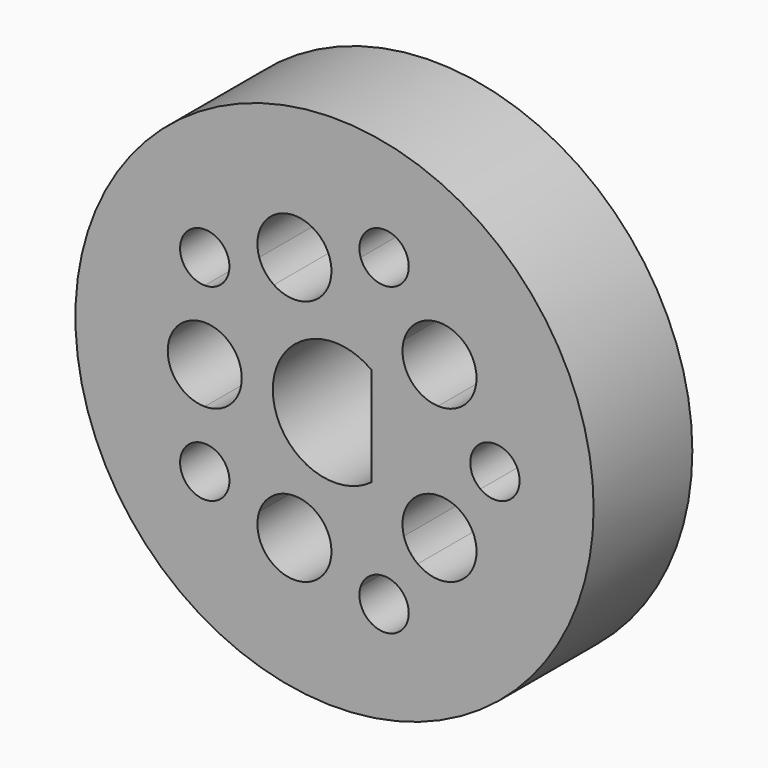
from build123d import *

# Parameters (mm, degrees)
F0_R     = 10.5
F1_DEPTH = 5


# Not quite as in the source:
# - a feature names something its author has since deleted; it is built from what else it names


with BuildPart() as f1:
    # F0 (on Front) → F1 (new body)
    with BuildSketch(Plane.XZ):
        Circle(F0_R)
        with BuildLine():
            Line((-6.1874431518, -2.6427799437), (-5.2586104634, -1.91030207))
            Line((-5.2586104634, -1.91030207), (-5.2586104634, -1.5))
            ThreePointArc((-5.2586104634, -1.5), (-6.7586104634, 0), (-5.2586104634, 1.5))
            Line((-5.2586104634, 1.5), (-5.2586104634, 1.91030207))
            Line((-5.2586104634, 1.91030207), (-6.1874431518, 2.6427799437))
            ThreePointArc((-6.1874431518, 2.6427799437), (-6.472135955, 4.7022820183), (-4.4254581722, 5.0679442137))
            Line((-4.4254581722, 5.0679442137), (-3.4418052317, 4.4109199439))
            Line((-3.4418052317, 4.4109199439), (-3.0515847744, 4.5377102563))
            ThreePointArc((-3.0515847744, 4.5377102563), (-2.0885254916, 6.4278205224), (-0.1984152256, 5.4647612395))
            Line((-0.1984152256, 5.4647612395), (0.1918052317, 5.5915515519))
            Line((0.1918052317, 5.5915515519), (0.601408001, 6.7012720437))
            ThreePointArc((0.601408001, 6.7012720437), (2.2724250824, 7.6584857382), (3.5086104634, 6.1818673559))
            ThreePointArc((3.5086104634, 6.1818673559), (3.4944811986, 5.976469794), (3.4523595855, 5.7749417209))
            Line((3.4523595855, 5.7749417209), (3.1314578476, 4.6364005169))
            Line((3.1314578476, 4.6364005169), (3.3726273533, 4.3044591695))
            ThreePointArc((3.3726273533, 4.3044591695), (4.9352909813, 4.4274434642), (5.7543052317, 3.090933678))
            ThreePointArc((5.7543052317, 3.090933678), (5.590815018, 2.4099479283), (5.1359831102, 1.8774081864))
            Line((5.1359831102, 1.8774081864), (5.3771526159, 1.545466839))
            Line((5.3771526159, 1.545466839), (6.5591337375, 1.4988339471))
            ThreePointArc((6.5591337375, 1.4988339471), (7.5813650184, 1.0395430231), (8, 0))
            ThreePointArc((8, 0), (7.5813650184, -1.0395430231), (6.5591337375, -1.4988339471))
            Line((6.5591337375, -1.4988339471), (5.3771526159, -1.545466839))
            Line((5.3771526159, -1.545466839), (5.1359831102, -1.8774081864))
            ThreePointArc((5.1359831102, -1.8774081864), (5.590815018, -2.4099479283), (5.7543052317, -3.090933678))
            ThreePointArc((5.7543052317, -3.090933678), (4.9352909813, -4.4274434642), (3.3726273533, -4.3044591695))
            Line((3.3726273533, -4.3044591695), (3.1314578476, -4.6364005169))
            Line((3.1314578476, -4.6364005169), (3.4523595855, -5.7749417209))
            ThreePointArc((3.4523595855, -5.7749417209), (3.4944811986, -5.976469794), (3.5086104634, -6.1818673559))
            ThreePointArc((3.5086104634, -6.1818673559), (2.2724250824, -7.6584857382), (0.601408001, -6.7012720437))
            Line((0.601408001, -6.7012720437), (0.1918052317, -5.5915515519))
            Line((0.1918052317, -5.5915515519), (-0.1984152256, -5.4647612395))
            ThreePointArc((-0.1984152256, -5.4647612395), (-2.0885254916, -6.4278205224), (-3.0515847744, -4.5377102563))
            Line((-3.0515847744, -4.5377102563), (-3.4418052317, -4.4109199439))
            Line((-3.4418052317, -4.4109199439), (-4.4254581722, -5.0679442137))
            ThreePointArc((-4.4254581722, -5.0679442137), (-6.472135955, -4.7022820183), (-6.1874431518, -2.6427799437))
        make_face(mode=Mode.SUBTRACT)
        with BuildLine():
            Line((-5.2586104634, -1.91030207), (-5.2586104634, -2.3206041399))
            ThreePointArc((-5.2586104634, -2.3206041399), (-4.1979502917, -2.7599439681), (-3.7586104634, -3.8206041399))
            ThreePointArc((-3.7586104634, -3.8206041399), (-3.7770779525, -4.0552558375), (-3.832025689, -4.2841296315))
            Line((-3.832025689, -4.2841296315), (-3.4418052317, -4.4109199439))
            Line((-3.4418052317, -4.4109199439), (-2.4581522912, -3.7538956741))
            ThreePointArc((-2.4581522912, -3.7538956741), (-1.1614745084, -3.5746509735), (-0.2177975376, -4.4818310601))
            Line((-0.2177975376, -4.4818310601), (0.1918052317, -5.5915515519))
            Line((0.1918052317, -5.5915515519), (0.582025689, -5.7183418644))
            ThreePointArc((0.582025689, -5.7183418644), (1.5450849719, -4.7552825815), (2.8902883419, -4.9683418644))
            Line((2.8902883419, -4.9683418644), (3.1314578476, -4.6364005169))
            Line((3.1314578476, -4.6364005169), (2.8105561096, -3.497859313))
            ThreePointArc((2.8105561096, -3.497859313), (3.0407797402, -2.2092557995), (4.1951714942, -1.5920997308))
            Line((4.1951714942, -1.5920997308), (5.3771526159, -1.545466839))
            Line((5.3771526159, -1.545466839), (5.6183221216, -1.2135254916))
            ThreePointArc((5.6183221216, -1.2135254916), (5, 0), (5.6183221216, 1.2135254916))
            Line((5.6183221216, 1.2135254916), (5.3771526159, 1.545466839))
            Line((5.3771526159, 1.545466839), (4.1951714942, 1.5920997308))
            ThreePointArc((4.1951714942, 1.5920997308), (3.0407797402, 2.2092557995), (2.8105561096, 3.497859313))
            Line((2.8105561096, 3.497859313), (3.1314578476, 4.6364005169))
            Line((3.1314578476, 4.6364005169), (2.8902883419, 4.9683418644))
            ThreePointArc((2.8902883419, 4.9683418644), (1.5450849719, 4.7552825815), (0.582025689, 5.7183418644))
            Line((0.582025689, 5.7183418644), (0.1918052317, 5.5915515519))
            Line((0.1918052317, 5.5915515519), (-0.2177975376, 4.4818310601))
            ThreePointArc((-0.2177975376, 4.4818310601), (-1.1614745084, 3.5746509735), (-2.4581522912, 3.7538956741))
            Line((-2.4581522912, 3.7538956741), (-3.4418052317, 4.4109199439))
            Line((-3.4418052317, 4.4109199439), (-3.832025689, 4.2841296315))
            ThreePointArc((-3.832025689, 4.2841296315), (-3.7770779525, 4.0552558375), (-3.7586104634, 3.8206041399))
            ThreePointArc((-3.7586104634, 3.8206041399), (-4.1979502917, 2.7599439681), (-5.2586104634, 2.3206041399))
            Line((-5.2586104634, 2.3206041399), (-5.2586104634, 1.91030207))
            Line((-5.2586104634, 1.91030207), (-4.3297777751, 1.1778241962))
            ThreePointArc((-4.3297777751, 1.1778241962), (-3.9089347556, 0.6545039983), (-3.7586104634, 0))
            ThreePointArc((-3.7586104634, 0), (-3.9089347556, -0.6545039983), (-4.3297777751, -1.1778241962))
            Line((-4.3297777751, -1.1778241962), (-5.2586104634, -1.91030207))
        make_face()
        with BuildLine():
            ThreePointArc((1.5, 2), (2.2360679775, 1.1180339887), (2.5, 0))
            ThreePointArc((2.5, 0), (2.2360679775, -1.1180339887), (1.5, -2))
            ThreePointArc((1.5, -2), (-2.5, 0), (1.5, 2))
        make_face(mode=Mode.SUBTRACT)
        with BuildLine():
            ThreePointArc((1.5, -2), (2.2360679775, -1.1180339887), (2.5, 0))
            ThreePointArc((2.5, 0), (2.2360679775, 1.1180339887), (1.5, 2))
            Line((1.5, 2), (1.5, -2))
        make_face()
        with BuildLine():
            ThreePointArc((-4.3075539471, -4.1296211343), (-6.0676274578, -4.4083893922), (-5.2586104634, -2.8206041399))
            Line((-5.2586104634, -2.8206041399), (-5.2586104634, -2.3206041399))
            ThreePointArc((-5.2586104634, -2.3206041399), (-5.7501710933, -2.403435079), (-6.1874431518, -2.6427799437))
            ThreePointArc((-6.1874431518, -2.6427799437), (-6.472135955, -4.7022820183), (-4.4254581722, -5.0679442137))
            ThreePointArc((-4.4254581722, -5.0679442137), (-4.0627031818, -4.7260354038), (-3.832025689, -4.2841296315))
            Line((-3.832025689, -4.2841296315), (-4.3075539471, -4.1296211343))
        make_face()
        with BuildLine():
            ThreePointArc((-6.1874431518, 2.6427799437), (-5.7501710933, 2.403435079), (-5.2586104634, 2.3206041399))
            Line((-5.2586104634, 2.3206041399), (-5.2586104634, 2.8206041399))
            ThreePointArc((-5.2586104634, 2.8206041399), (-6.0676274578, 4.4083893922), (-4.3075539471, 4.1296211343))
            Line((-4.3075539471, 4.1296211343), (-3.832025689, 4.2841296315))
            ThreePointArc((-3.832025689, 4.2841296315), (-4.0627031818, 4.7260354038), (-4.4254581722, 5.0679442137))
            ThreePointArc((-4.4254581722, 5.0679442137), (-6.472135955, 4.7022820183), (-6.1874431518, 2.6427799437))
        make_face()
        with BuildLine():
            Line((1.0575539471, -5.8728503615), (0.582025689, -5.7183418644))
            ThreePointArc((0.582025689, -5.7183418644), (0.508902005, -6.2114399724), (0.601408001, -6.7012720437))
            ThreePointArc((0.601408001, -6.7012720437), (2.2724250824, -7.6584857382), (3.5086104634, -6.1818673559))
            ThreePointArc((3.5086104634, -6.1818673559), (3.4944811986, -5.976469794), (3.4523595855, -5.7749417209))
            ThreePointArc((3.4523595855, -5.7749417209), (3.2392824408, -5.3242855906), (2.8902883419, -4.9683418644))
            Line((2.8902883419, -4.9683418644), (2.5963957157, -5.3728503615))
            ThreePointArc((2.5963957157, -5.3728503615), (2.8996169876, -5.7278768562), (3.0086104634, -6.1818673559))
            ThreePointArc((3.0086104634, -6.1818673559), (1.8521759984, -7.1695556965), (1.0575539471, -5.8728503615))
        make_face()
        with BuildLine():
            ThreePointArc((0.601408001, 6.7012720437), (0.508902005, 6.2114399724), (0.582025689, 5.7183418644))
            Line((0.582025689, 5.7183418644), (1.0575539471, 5.8728503615))
            ThreePointArc((1.0575539471, 5.8728503615), (1.8521759984, 7.1695556965), (3.0086104634, 6.1818673559))
            ThreePointArc((3.0086104634, 6.1818673559), (2.8996169876, 5.7278768562), (2.5963957157, 5.3728503615))
            Line((2.5963957157, 5.3728503615), (2.8902883419, 4.9683418644))
            ThreePointArc((2.8902883419, 4.9683418644), (3.2392824408, 5.3242855906), (3.4523595855, 5.7749417209))
            ThreePointArc((3.4523595855, 5.7749417209), (3.4944811986, 5.976469794), (3.5086104634, 6.1818673559))
            ThreePointArc((3.5086104634, 6.1818673559), (2.2724250824, 7.6584857382), (0.601408001, 6.7012720437))
        make_face()
        with BuildLine():
            Line((5.9122147477, -0.8090169944), (5.6183221216, -1.2135254916))
            ThreePointArc((5.6183221216, -1.2135254916), (6.0646898294, -1.435445943), (6.5591337375, -1.4988339471))
            ThreePointArc((6.5591337375, -1.4988339471), (7.5813650184, -1.0395430231), (8, 0))
            ThreePointArc((8, 0), (7.5813650184, 1.0395430231), (6.5591337375, 1.4988339471))
            ThreePointArc((6.5591337375, 1.4988339471), (6.0646898294, 1.435445943), (5.6183221216, 1.2135254916))
            Line((5.6183221216, 1.2135254916), (5.9122147477, 0.8090169944))
            ThreePointArc((5.9122147477, 0.8090169944), (6.9539904997, 0.8910065242), (7.5, 0))
            ThreePointArc((7.5, 0), (6.9539904997, -0.8910065242), (5.9122147477, -0.8090169944))
        make_face()
        with BuildLine():
            Line((-5.2586104634, -2.3206041399), (-5.2586104634, -2.8206041399))
            ThreePointArc((-5.2586104634, -2.8206041399), (-4.5515036823, -3.1134973587), (-4.2586104634, -3.8206041399))
            ThreePointArc((-4.2586104634, -3.8206041399), (-4.2709221228, -3.9770386049), (-4.3075539471, -4.1296211343))
            Line((-4.3075539471, -4.1296211343), (-3.832025689, -4.2841296315))
            ThreePointArc((-3.832025689, -4.2841296315), (-3.7770779525, -4.0552558375), (-3.7586104634, -3.8206041399))
            ThreePointArc((-3.7586104634, -3.8206041399), (-4.1979502917, -2.7599439681), (-5.2586104634, -2.3206041399))
        make_face()
        with BuildLine():
            Line((-5.2586104634, 2.8206041399), (-5.2586104634, 2.3206041399))
            ThreePointArc((-5.2586104634, 2.3206041399), (-4.1979502917, 2.7599439681), (-3.7586104634, 3.8206041399))
            ThreePointArc((-3.7586104634, 3.8206041399), (-3.7770779525, 4.0552558375), (-3.832025689, 4.2841296315))
            Line((-3.832025689, 4.2841296315), (-4.3075539471, 4.1296211343))
            ThreePointArc((-4.3075539471, 4.1296211343), (-4.2709221228, 3.9770386049), (-4.2586104634, 3.8206041399))
            ThreePointArc((-4.2586104634, 3.8206041399), (-4.5515036823, 3.1134973587), (-5.2586104634, 2.8206041399))
        make_face()
        with BuildLine():
            ThreePointArc((2.8902883419, -4.9683418644), (1.5450849719, -4.7552825815), (0.582025689, -5.7183418644))
            Line((0.582025689, -5.7183418644), (1.0575539471, -5.8728503615))
            ThreePointArc((1.0575539471, -5.8728503615), (1.6995934691, -5.2308108396), (2.5963957157, -5.3728503615))
            Line((2.5963957157, -5.3728503615), (2.8902883419, -4.9683418644))
        make_face()
        with BuildLine():
            Line((1.0575539471, 5.8728503615), (0.582025689, 5.7183418644))
            ThreePointArc((0.582025689, 5.7183418644), (1.5450849719, 4.7552825815), (2.8902883419, 4.9683418644))
            Line((2.8902883419, 4.9683418644), (2.5963957157, 5.3728503615))
            ThreePointArc((2.5963957157, 5.3728503615), (1.6995934691, 5.2308108396), (1.0575539471, 5.8728503615))
        make_face()
        with BuildLine():
            ThreePointArc((5.6183221216, 1.2135254916), (5, 0), (5.6183221216, -1.2135254916))
            Line((5.6183221216, -1.2135254916), (5.9122147477, -0.8090169944))
            ThreePointArc((5.9122147477, -0.8090169944), (5.5, 0), (5.9122147477, 0.8090169944))
            Line((5.9122147477, 0.8090169944), (5.6183221216, 1.2135254916))
        make_face()
        with BuildLine():
            ThreePointArc((-6.1874431518, -2.6427799437), (-5.7501710933, -2.403435079), (-5.2586104634, -2.3206041399))
            Line((-5.2586104634, -2.3206041399), (-5.2586104634, -1.91030207))
            Line((-5.2586104634, -1.91030207), (-6.1874431518, -2.6427799437))
        make_face()
        with BuildLine():
            Line((-3.4418052317, -4.4109199439), (-3.832025689, -4.2841296315))
            ThreePointArc((-3.832025689, -4.2841296315), (-4.0627031818, -4.7260354038), (-4.4254581722, -5.0679442137))
            Line((-4.4254581722, -5.0679442137), (-3.4418052317, -4.4109199439))
        make_face()
        with BuildLine():
            Line((-5.2586104634, -1.5), (-5.2586104634, -1.91030207))
            Line((-5.2586104634, -1.91030207), (-4.3297777751, -1.1778241962))
            ThreePointArc((-4.3297777751, -1.1778241962), (-4.7670498335, -1.4171690609), (-5.2586104634, -1.5))
        make_face()
        with BuildLine():
            Line((-2.4581522912, -3.7538956741), (-3.4418052317, -4.4109199439))
            Line((-3.4418052317, -4.4109199439), (-3.0515847744, -4.5377102563))
            ThreePointArc((-3.0515847744, -4.5377102563), (-2.8209072816, -4.095804484), (-2.4581522912, -3.7538956741))
        make_face()
        with BuildLine():
            Line((-5.2586104634, 1.91030207), (-5.2586104634, 1.5))
            ThreePointArc((-5.2586104634, 1.5), (-4.7670498335, 1.4171690609), (-4.3297777751, 1.1778241962))
            Line((-4.3297777751, 1.1778241962), (-5.2586104634, 1.91030207))
        make_face()
        with BuildLine():
            ThreePointArc((-0.125, -5.0012357479), (-0.1434674891, -5.2358874455), (-0.1984152256, -5.4647612395))
            Line((-0.1984152256, -5.4647612395), (0.1918052317, -5.5915515519))
            Line((0.1918052317, -5.5915515519), (-0.2177975376, -4.4818310601))
            ThreePointArc((-0.2177975376, -4.4818310601), (-0.1483816177, -4.737421129), (-0.125, -5.0012357479))
        make_face()
        with BuildLine():
            Line((-6.1874431518, 2.6427799437), (-5.2586104634, 1.91030207))
            Line((-5.2586104634, 1.91030207), (-5.2586104634, 2.3206041399))
            ThreePointArc((-5.2586104634, 2.3206041399), (-5.7501710933, 2.403435079), (-6.1874431518, 2.6427799437))
        make_face()
        with BuildLine():
            Line((0.582025689, -5.7183418644), (0.1918052317, -5.5915515519))
            Line((0.1918052317, -5.5915515519), (0.601408001, -6.7012720437))
            ThreePointArc((0.601408001, -6.7012720437), (0.508902005, -6.2114399724), (0.582025689, -5.7183418644))
        make_face()
        with BuildLine():
            Line((-3.4418052317, 4.4109199439), (-4.4254581722, 5.0679442137))
            ThreePointArc((-4.4254581722, 5.0679442137), (-4.0627031818, 4.7260354038), (-3.832025689, 4.2841296315))
            Line((-3.832025689, 4.2841296315), (-3.4418052317, 4.4109199439))
        make_face()
        with BuildLine():
            Line((3.1314578476, -4.6364005169), (2.8902883419, -4.9683418644))
            ThreePointArc((2.8902883419, -4.9683418644), (3.2392824408, -5.3242855906), (3.4523595855, -5.7749417209))
            Line((3.4523595855, -5.7749417209), (3.1314578476, -4.6364005169))
        make_face()
        with BuildLine():
            Line((-3.0515847744, 4.5377102563), (-3.4418052317, 4.4109199439))
            Line((-3.4418052317, 4.4109199439), (-2.4581522912, 3.7538956741))
            ThreePointArc((-2.4581522912, 3.7538956741), (-2.8209072816, 4.095804484), (-3.0515847744, 4.5377102563))
        make_face()
        with BuildLine():
            Line((2.8105561096, -3.497859313), (3.1314578476, -4.6364005169))
            Line((3.1314578476, -4.6364005169), (3.3726273533, -4.3044591695))
            ThreePointArc((3.3726273533, -4.3044591695), (3.0236332544, -3.9485154433), (2.8105561096, -3.497859313))
        make_face()
        with BuildLine():
            Line((0.1918052317, 5.5915515519), (-0.1984152256, 5.4647612395))
            ThreePointArc((-0.1984152256, 5.4647612395), (-0.1434674891, 5.2358874455), (-0.125, 5.0012357479))
            ThreePointArc((-0.125, 5.0012357479), (-0.1483816177, 4.737421129), (-0.2177975376, 4.4818310601))
            Line((-0.2177975376, 4.4818310601), (0.1918052317, 5.5915515519))
        make_face()
        with BuildLine():
            ThreePointArc((4.1951714942, -1.5920997308), (4.6896154024, -1.6554877349), (5.1359831102, -1.8774081864))
            Line((5.1359831102, -1.8774081864), (5.3771526159, -1.545466839))
            Line((5.3771526159, -1.545466839), (4.1951714942, -1.5920997308))
        make_face()
        with BuildLine():
            Line((0.601408001, 6.7012720437), (0.1918052317, 5.5915515519))
            Line((0.1918052317, 5.5915515519), (0.582025689, 5.7183418644))
            ThreePointArc((0.582025689, 5.7183418644), (0.508902005, 6.2114399724), (0.601408001, 6.7012720437))
        make_face()
        with BuildLine():
            Line((5.6183221216, -1.2135254916), (5.3771526159, -1.545466839))
            Line((5.3771526159, -1.545466839), (6.5591337375, -1.4988339471))
            ThreePointArc((6.5591337375, -1.4988339471), (6.0646898294, -1.435445943), (5.6183221216, -1.2135254916))
        make_face()
        with BuildLine():
            ThreePointArc((3.4523595855, 5.7749417209), (3.2392824408, 5.3242855906), (2.8902883419, 4.9683418644))
            Line((2.8902883419, 4.9683418644), (3.1314578476, 4.6364005169))
            Line((3.1314578476, 4.6364005169), (3.4523595855, 5.7749417209))
        make_face()
        with BuildLine():
            Line((5.3771526159, 1.545466839), (5.6183221216, 1.2135254916))
            ThreePointArc((5.6183221216, 1.2135254916), (6.0646898294, 1.435445943), (6.5591337375, 1.4988339471))
            Line((6.5591337375, 1.4988339471), (5.3771526159, 1.545466839))
        make_face()
        with BuildLine():
            Line((3.3726273533, 4.3044591695), (3.1314578476, 4.6364005169))
            Line((3.1314578476, 4.6364005169), (2.8105561096, 3.497859313))
            ThreePointArc((2.8105561096, 3.497859313), (3.0236332544, 3.9485154433), (3.3726273533, 4.3044591695))
        make_face()
        with BuildLine():
            Line((4.1951714942, 1.5920997308), (5.3771526159, 1.545466839))
            Line((5.3771526159, 1.545466839), (5.1359831102, 1.8774081864))
            ThreePointArc((5.1359831102, 1.8774081864), (4.6896154024, 1.6554877349), (4.1951714942, 1.5920997308))
        make_face()
    extrude(amount=F1_DEPTH)


solid = f1.part
